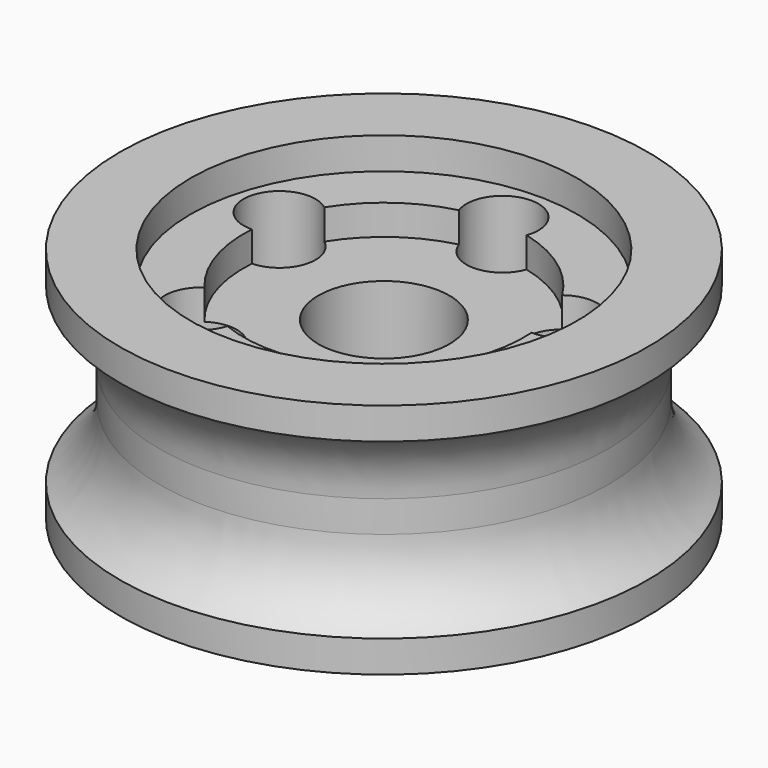
from build123d import *

# Parameters (mm, degrees)
F1_FACE_R   = 34.7840711474
F1_FACE_R_2 = 25.2269001212
F3_R        = 6.4772859213
F4_DEPTH    = 236.4


# Not quite as in the source:
# - a fillet or chamfer that OpenCascade refuses, or shapes differently, is made with other operations: its cross-section is extruded or revolved along the edge and cut away or added


with BuildPart() as f1:
    # F0 (on Front) → F1 (revolve)
    with BuildSketch(Plane.XZ):
        Polygon((-11.804982787, 11.1373364925), (-11.804982787, 21.3137716055), (-11.804982787, 31.4902067184), (-25.2269001212, 31.4902067184), (-25.2269001212, 36.9160883129), (-34.7840711474, 36.9160883129), (-34.7840711474, 42.627543211), (-47.5015656557, 42.627543211), (-47.5015656557, 36.9160883129), (-40.3622516897, 36.9160883129), (-40.3622516897, 21.3137716055), (-40.3622516897, 5.7114548981), (-47.5015656557, 5.7114548981), (-47.5015656557, 0), (-34.7840711474, 0), (-34.7840711474, 5.7114548981), (-25.2269001212, 5.7114548981), (-25.2269001212, 11.1373364925), align=None)
    revolve(axis=Axis((0, 0, 40.0708690286), (0, 0, 1)))

    # F2: fillet of radius 15 on 3 edges, made by hand

    # F2_s1 → F2_t2 (revolve)
    with BuildSketch(Plane.XZ):
        with BuildLine():
            ThreePointArc((-47.5015656557, 36.9160883129), (-42.2681635101, 31.4581714397), (-40.3622516897, 24.1407364557))
            Line((-40.3622516897, 24.1407364557), (-40.0622516897, 24.1407364557))
            Line((-40.0622516897, 24.1407364557), (-40.0622516897, 36.9160883129))
            Line((-40.0622516897, 36.9160883129), (-40.3622516897, 37.2160883129))
            ThreePointArc((-40.3622516897, 37.2160883129), (-43.9319086727, 37.2160883129), (-47.344351935, 37.17159535))
            Line((-47.344351935, 37.17159535), (-47.5015656557, 36.9160883129))
        make_face()
    revolve(axis=Axis((0, 0, 36.9160883129), (0, 0, 1)))

    # F2_s3 → F2_t4 (revolve)
    with BuildSketch(Plane.XZ):
        with BuildLine():
            ThreePointArc((-40.3622516897, 18.4868067553), (-42.2681635101, 11.1693717713), (-47.5015656557, 5.7114548981))
            Line((-47.5015656557, 5.7114548981), (-47.344351935, 5.455947861))
            ThreePointArc((-47.344351935, 5.455947861), (-43.9319086727, 5.4114548981), (-40.3622516897, 5.4114548981))
            Line((-40.3622516897, 5.4114548981), (-40.0622516897, 5.7114548981))
            Line((-40.0622516897, 5.7114548981), (-40.0622516897, 18.4868067553))
            Line((-40.0622516897, 18.4868067553), (-40.3622516897, 18.4868067553))
        make_face()
    revolve(axis=Axis((0, 0, 5.7114548981), (0, 0, 1)))

    # F1_face (on face) + F3 (on Top) → F4 (cut)
    with BuildSketch(Plane.XY.offset(36.9160883129)):
        Circle(F1_FACE_R)
        Circle(F1_FACE_R_2, mode=Mode.SUBTRACT)
    with BuildSketch(Plane.XY):
        with Locations((0, 26.6724559541)):
            Circle(F3_R)
        with Locations((-25.3670130407, 8.2422421715)):
            Circle(F3_R)
        with Locations((-15.6776762522, -21.5784701486)):
            Circle(F3_R)
        with Locations((15.6776762522, -21.5784701486)):
            Circle(F3_R)
        with Locations((25.3670130407, 8.2422421715)):
            Circle(F3_R)
    extrude(amount=F4_DEPTH, mode=Mode.SUBTRACT)


solid = f1.part
